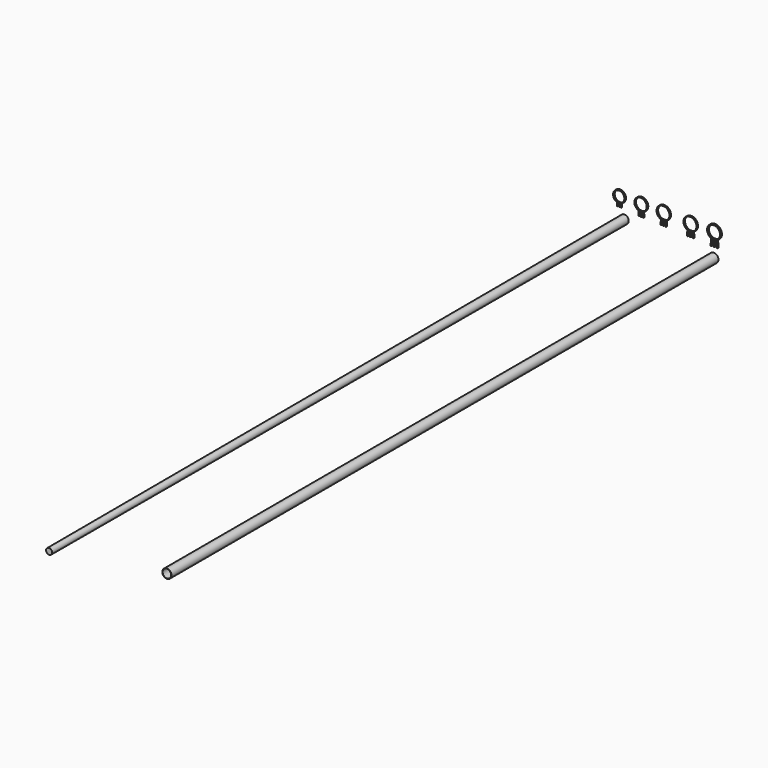
from build123d import *

# Parameters (mm, degrees)
F0_R      = 2.62636
F1_DEPTH  = 391.16
F2_R      = 2.4545174693
F3_DEPTH  = 27.2034
F4_R      = 2.45491
F5_DEPTH  = 411.48
F5_TAPER  = 0.1
F6_R      = 3.4566135919
F7_DEPTH  = 0.762
F8_DEPTH  = 0.762
F9_R      = 3.5884802504
F10_DEPTH = 0.762
F11_R     = 3.5392622184
F12_DEPTH = 0.762
F13_R     = 3.3722563351
F14_DEPTH = 0.762
F15_R     = 3.0524378361
F16_DEPTH = 0.762


# Not quite as in the source:
# - a feature names something its author has since deleted; it is built from what else it names


with BuildPart() as f1:
    # F0 (on Front) → F1 (new body)
    with BuildSketch(Plane.XZ):
        with Locations((33.3854705095, 22.1610423177)):
            Circle(F0_R)
    extrude(amount=F1_DEPTH)

    # F2 (on face) → F3 (cut)
    with BuildSketch(Plane.XZ.offset(391.16)):
        with Locations((33.3854705095, 22.1610423177)):
            Circle(F2_R)
    extrude(amount=-F3_DEPTH, mode=Mode.SUBTRACT)


with BuildPart() as f5:
    # F4 (on Front) → F5 (new body)
    with BuildSketch(Plane.XZ):
        with Locations((-17.7624952048, 24.9722655863)):
            Circle(F4_R)
    extrude(amount=F5_DEPTH, taper=F5_TAPER)


with BuildPart() as f7:
    # F6 (on Front) → F7 (new body)
    with BuildSketch(Plane.XZ):
        with BuildLine():
            ThreePointArc((35.7715754489, 32.0952818217), (37.4092534584, 33.5469125299), (38.0179269561, 35.6489918694))
            ThreePointArc((38.0179269561, 35.6489918694), (31.9817014824, 38.974464506), (32.3959861948, 32.0952818217))
            ThreePointArc((32.3959861948, 32.0952818217), (32.6536943465, 31.9839736594), (32.9186837167, 31.8913257664))
            ThreePointArc((32.9186837167, 31.8913257664), (33.3814730836, 31.7780398357), (33.8545631583, 31.7215289391))
            ThreePointArc((33.8545631583, 31.7215289391), (34.0837808218, 31.7148457351), (34.3129984853, 31.7215289391))
            ThreePointArc((34.3129984853, 31.7215289391), (34.817521405, 31.783874722), (35.3097929415, 31.91075698))
            ThreePointArc((35.3097929415, 31.91075698), (35.5436026581, 31.9957158036), (35.7715754489, 32.0952818217))
        make_face()
        with Locations((34.0837808218, 35.6489918694)):
            Circle(F6_R, mode=Mode.SUBTRACT)
    extrude(amount=F7_DEPTH)

    # F6 (on Front) → F8 (join)
    with BuildSketch(Plane.XZ):
        with BuildLine():
            ThreePointArc((35.7715754489, 32.0952818217), (37.4092534584, 33.5469125299), (38.0179269561, 35.6489918694))
            ThreePointArc((38.0179269561, 35.6489918694), (31.9817014824, 38.974464506), (32.3959861948, 32.0952818217))
            ThreePointArc((32.3959861948, 32.0952818217), (32.6536943465, 31.9839736594), (32.9186837167, 31.8913257664))
            ThreePointArc((32.9186837167, 31.8913257664), (33.3814730836, 31.7780398357), (33.8545631583, 31.7215289391))
            ThreePointArc((33.8545631583, 31.7215289391), (34.0837808218, 31.7148457351), (34.3129984853, 31.7215289391))
            ThreePointArc((34.3129984853, 31.7215289391), (34.817521405, 31.783874722), (35.3097929415, 31.91075698))
            ThreePointArc((35.3097929415, 31.91075698), (35.5436026581, 31.9957158036), (35.7715754489, 32.0952818217))
        make_face()
        with Locations((34.0837808218, 35.6489918694)):
            Circle(F6_R, mode=Mode.SUBTRACT)
        with BuildLine():
            ThreePointArc((32.9186837167, 31.8913257664), (32.6536943465, 31.9839736594), (32.3959861948, 32.0952818217))
            Line((32.3959861948, 32.0952818217), (32.1424752474, 28.2143242631))
            Line((32.1424752474, 28.2143242631), (32.6762180922, 28.1794592453))
            Line((32.6762180922, 28.1794592453), (32.9186837167, 31.8913257664))
        make_face()
        with BuildLine():
            ThreePointArc((34.3129984853, 31.7215289391), (34.0837808218, 31.7148457351), (33.8545631583, 31.7215289391))
            Line((33.8545631583, 31.7215289391), (33.8545631583, 28.2143242631))
            Line((33.8545631583, 28.2143242631), (34.3129984853, 28.2143242631))
            Line((34.3129984853, 28.2143242631), (34.3129984853, 31.7215289391))
        make_face()
        with BuildLine():
            Line((36.1872240901, 28.2143242631), (35.7715754489, 32.0952818217))
            ThreePointArc((35.7715754489, 32.0952818217), (35.5436026581, 31.9957158036), (35.3097929415, 31.91075698))
            Line((35.3097929415, 31.91075698), (35.5512574315, 28.2143242631))
            Line((35.5512574315, 28.2143242631), (36.1872240901, 28.2143242631))
        make_face()
    extrude(amount=F8_DEPTH)


with BuildPart() as f10:
    # F9 (on Front) → F10 (new body)
    with BuildSketch(Plane.XZ):
        with BuildLine():
            ThreePointArc((22.1319308048, 31.8462318345), (23.7415235219, 33.2722886782), (24.3397960437, 35.3378386838))
            ThreePointArc((24.3397960437, 35.3378386838), (18.4094296981, 38.6043825019), (18.8180286027, 31.8462318345))
            ThreePointArc((18.8180286027, 31.8462318345), (19.0471481942, 31.7464458452), (19.282237764, 31.6616760097))
            ThreePointArc((19.282237764, 31.6616760097), (19.7223206629, 31.5470195494), (20.1728250831, 31.4848518))
            ThreePointArc((20.1728250831, 31.4848518), (20.4000461089, 31.473748843), (20.6275267627, 31.476034088))
            ThreePointArc((20.6275267627, 31.476034088), (21.1896761466, 31.5396793486), (21.736511169, 31.6847107496))
            ThreePointArc((21.736511169, 31.6847107496), (21.9364540921, 31.7600044292), (22.1319308048, 31.8462318345))
        make_face()
        with Locations((20.4749797037, 35.3378386838)):
            Circle(F9_R, mode=Mode.SUBTRACT)
        with BuildLine():
            Line((22.267555818, 28.7543646982), (22.1319308048, 31.8462318345))
            ThreePointArc((22.1319308048, 31.8462318345), (21.9364540921, 31.7600044292), (21.736511169, 31.6847107496))
            Line((21.736511169, 31.6847107496), (21.8658240366, 28.7367426996))
            Line((21.8658240366, 28.7367426996), (22.267555818, 28.7543646982))
        make_face()
        with BuildLine():
            ThreePointArc((20.6275267627, 31.476034088), (20.4000461089, 31.473748843), (20.1728250831, 31.4848518))
            Line((20.1728250831, 31.4848518), (20.1728250831, 28.7543646982))
            Line((20.1728250831, 28.7543646982), (20.6275267627, 28.7543646982))
            Line((20.6275267627, 28.7543646982), (20.6275267627, 31.476034088))
        make_face()
        with BuildLine():
            ThreePointArc((19.282237764, 31.6616760097), (19.0471481942, 31.7464458452), (18.8180286027, 31.8462318345))
            Line((18.8180286027, 31.8462318345), (18.6983123422, 28.7543646982))
            Line((18.6983123422, 28.7543646982), (19.1689618492, 28.7361412764))
            Line((19.1689618492, 28.7361412764), (19.282237764, 31.6616760097))
        make_face()
    extrude(amount=F10_DEPTH)


with BuildPart() as f12:
    # F11 (on Front) → F12 (new body)
    with BuildSketch(Plane.XZ):
        with BuildLine():
            ThreePointArc((6.4378347425, 32.2904881093), (8.2090963798, 33.6979702133), (8.8772032465, 35.8594527775))
            ThreePointArc((8.8772032465, 35.8594527775), (2.8852154776, 39.0218511155), (3.6555613411, 32.2904881093))
            ThreePointArc((3.6555613411, 32.2904881093), (3.7886138591, 32.2414430605), (3.9233905263, 32.1973563357))
            ThreePointArc((3.9233905263, 32.1973563357), (4.3837529644, 32.0867516301), (4.8542437144, 32.0337853253))
            ThreePointArc((4.8542437144, 32.0337853253), (5.0656146513, 32.0289942821), (5.2769279587, 32.0358727393))
            ThreePointArc((5.2769279587, 32.0358727393), (5.6726558311, 32.0804387567), (6.0616182074, 32.165849228))
            ThreePointArc((6.0616182074, 32.165849228), (6.2513395336, 32.223299728), (6.4378347425, 32.2904881093))
        make_face()
        with Locations((5.0466980418, 35.8594527775)):
            Circle(F11_R, mode=Mode.SUBTRACT)
        with BuildLine():
            ThreePointArc((5.2769279587, 32.0358727393), (5.0656146513, 32.0289942821), (4.8542437144, 32.0337853253))
            Line((4.8542437144, 32.0337853253), (4.8542437144, 29.4231642021))
            Line((4.8542437144, 29.4231642021), (5.2769279587, 29.4231642021))
            Line((5.2769279587, 29.4231642021), (5.2769279587, 32.0358727393))
        make_face()
        with BuildLine():
            ThreePointArc((3.9233905263, 32.1973563357), (3.7886138591, 32.2414430605), (3.6555613411, 32.2904881093))
            Line((3.6555613411, 32.2904881093), (3.5838247277, 29.4231642021))
            Line((3.5838247277, 29.4231642021), (3.9233905263, 29.4231642021))
            Line((3.9233905263, 29.4231642021), (3.9233905263, 32.1973563357))
        make_face()
        with BuildLine():
            Line((6.6511374898, 29.4231642021), (6.4378347425, 32.2904881093))
            ThreePointArc((6.4378347425, 32.2904881093), (6.2513395336, 32.223299728), (6.0616182074, 32.165849228))
            Line((6.0616182074, 32.165849228), (6.2677705127, 29.3946451955))
            Line((6.2677705127, 29.3946451955), (6.6511374898, 29.4231642021))
        make_face()
    extrude(amount=F12_DEPTH)


with BuildPart() as f14:
    # F13 (on Front) → F14 (new body)
    with BuildSketch(Plane.XZ):
        with BuildLine():
            ThreePointArc((-6.5058638968, 32.5024286839), (-4.7653563145, 33.8496335486), (-4.1064509287, 35.9496743303))
            ThreePointArc((-4.1064509287, 35.9496743303), (-9.882533595, 38.9668108291), (-9.0591217298, 32.5024286839))
            ThreePointArc((-9.0591217298, 32.5024286839), (-8.8648672093, 32.4365916947), (-8.667243059, 32.3816915753))
            ThreePointArc((-8.667243059, 32.3816915753), (-8.2977321652, 32.3099198952), (-7.9228188843, 32.2763117657))
            ThreePointArc((-7.9228188843, 32.2763117657), (-7.7003077273, 32.2745512645), (-7.4780977065, 32.2862568607))
            ThreePointArc((-7.4780977065, 32.2862568607), (-7.1536774965, 32.3278135882), (-6.8342351877, 32.3980421122))
            ThreePointArc((-6.8342351877, 32.3980421122), (-6.6688258207, 32.4463859084), (-6.5058638968, 32.5024286839))
        make_face()
        with Locations((-7.7824928133, 35.9496743303)):
            Circle(F13_R, mode=Mode.SUBTRACT)
        with BuildLine():
            ThreePointArc((-7.4780977065, 32.2862568607), (-7.7003077273, 32.2745512645), (-7.9228188843, 32.2763117657))
            Line((-7.9228188843, 32.2763117657), (-7.9228188843, 29.7263376413))
            Line((-7.9228188843, 29.7263376413), (-7.4780977065, 29.7263376413))
            Line((-7.4780977065, 29.7263376413), (-7.4780977065, 32.2862568607))
        make_face()
        with BuildLine():
            ThreePointArc((-8.667243059, 32.3816915753), (-8.8648672093, 32.4365916947), (-9.0591217298, 32.5024286839))
            Line((-9.0591217298, 32.5024286839), (-9.1820461676, 29.7263376413))
            Line((-9.1820461676, 29.7263376413), (-8.7855986065, 29.7087830681))
            Line((-8.7855986065, 29.7087830681), (-8.667243059, 32.3816915753))
        make_face()
        with BuildLine():
            Line((-6.3007362187, 29.7507625073), (-6.5058638968, 32.5024286839))
            ThreePointArc((-6.5058638968, 32.5024286839), (-6.6688258207, 32.4463859084), (-6.8342351877, 32.3980421122))
            Line((-6.8342351877, 32.3980421122), (-6.6350314361, 29.7258418966))
            Line((-6.6350314361, 29.7258418966), (-6.3007362187, 29.7507625073))
        make_face()
    extrude(amount=F14_DEPTH)


with BuildPart() as f16:
    # F15 (on Front) → F16 (new body)
    with BuildSketch(Plane.XZ):
        with BuildLine():
            ThreePointArc((-19.0943665325, 32.7215177714), (-17.4757935329, 33.9674438978), (-16.8625762084, 35.9157957603))
            ThreePointArc((-16.8625762084, 35.9157957603), (-22.2127485191, 38.7043988839), (-21.4344267806, 32.7215177714))
            ThreePointArc((-21.4344267806, 32.7215177714), (-21.3151586387, 32.6803233654), (-21.1944448053, 32.6435804859))
            ThreePointArc((-21.1944448053, 32.6435804859), (-20.7588494348, 32.5501013578), (-20.3147735447, 32.5143483433))
            ThreePointArc((-20.3147735447, 32.5143483433), (-20.1805968117, 32.5150076241), (-20.046550451, 32.5209577094))
            ThreePointArc((-20.046550451, 32.5209577094), (-19.686883893, 32.5633546543), (-19.3337626727, 32.643747052))
            ThreePointArc((-19.3337626727, 32.643747052), (-19.2133450428, 32.6804174414), (-19.0943665325, 32.7215177714))
        make_face()
        with Locations((-20.2643966565, 35.9157957603)):
            Circle(F15_R, mode=Mode.SUBTRACT)
        with BuildLine():
            ThreePointArc((-20.046550451, 32.5209577094), (-20.1805968117, 32.5150076241), (-20.3147735447, 32.5143483433))
            Line((-20.3147735447, 32.5143483433), (-20.3147735447, 30.6218452734))
            Line((-20.3147735447, 30.6218452734), (-20.046550451, 30.6218452734))
            Line((-20.046550451, 30.6218452734), (-20.046550451, 32.5209577094))
        make_face()
        with BuildLine():
            ThreePointArc((-21.1944448053, 32.6435804859), (-21.3151586387, 32.6803233654), (-21.4344267806, 32.7215177714))
            Line((-21.4344267806, 32.7215177714), (-21.4995890856, 30.7086575776))
            Line((-21.4995890856, 30.7086575776), (-21.2573379291, 30.7008151831))
            Line((-21.2573379291, 30.7008151831), (-21.1944448053, 32.6435804859))
        make_face()
        with BuildLine():
            Line((-19.011374563, 30.6218452734), (-19.0943665325, 32.7215177714))
            ThreePointArc((-19.0943665325, 32.7215177714), (-19.2133450428, 32.6804174414), (-19.3337626727, 32.643747052))
            Line((-19.3337626727, 32.643747052), (-19.2534664561, 30.612276313))
            Line((-19.2534664561, 30.612276313), (-19.011374563, 30.6218452734))
        make_face()
    extrude(amount=F16_DEPTH)


solid = Compound([f1.part, f5.part, f7.part, f10.part, f12.part, f14.part, f16.part])
